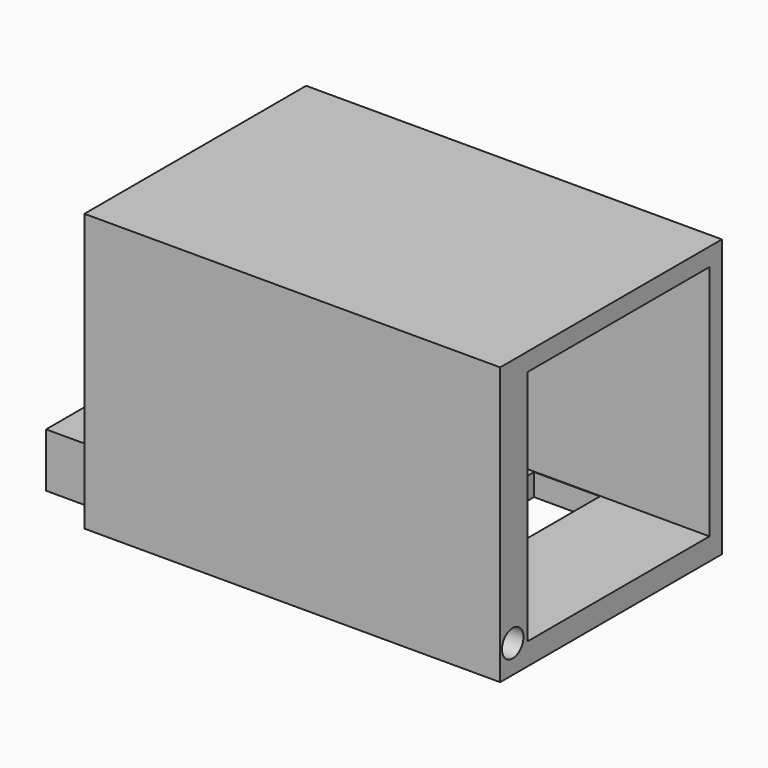
from build123d import *

# Parameters (mm, degrees)
F0_W         = 17.1955762447
F0_H         = 101.6
F0_W_2       = 121.0433589118
F0_W_3       = 14.1610648435
F1_DEPTH     = 101.6
F2_R         = 4.9213514136
F3_DEPTH     = 164.846
F4_W         = 24.1568293422
F4_H         = 84.1714516282
F5_DEPTH     = 19.812
F6_TEXT_SIZE = 13.509515499
F7_DEPTH     = 2.032
F8_DEPTH     = 111.506
F9_W         = 83.3843462169
F9_H         = 86.921655573
F10_DEPTH    = 139.954


# Not quite as in the source:
# - Text() gives the source's letters only with a copy of the font that has no kerning and outlines rounded to 1/6400 em; it was checked with that copy


with BuildPart() as f1:
    # F0 (on Top) → F1 (new body)
    with BuildSketch(Plane.XY):
        with Locations((73.6461340337, 72.8689902046)):
            Rectangle(F0_W, F0_H)
        with Locations((-9.634398388, 72.8689902046)):
            Rectangle(F0_W_2, F0_H)
        with Locations((57.9678134896, 72.8689902046)):
            Rectangle(F0_W_3, F0_H)
    extrude(amount=F1_DEPTH)

    # F2 (on face) → F3 (cut)
    with BuildSketch(Plane(origin=(-70.1560778439, 0, 0), x_dir=(0, -1, 0), z_dir=(-1, 0, 0))):
        with Locations((-27.8169699013, 10.2606434375)):
            Circle(F2_R)
    extrude(amount=-F3_DEPTH, mode=Mode.SUBTRACT)

    # F4 (on face) → F5 (cut)
    with BuildSketch(Plane(origin=(0, 0, 0), x_dir=(1, 0, 0), z_dir=(0, 0, -1))):
        with Locations((30.1983924583, -75.633931905)):
            Rectangle(F4_W, F4_H)
    extrude(amount=-F5_DEPTH, mode=Mode.SUBTRACT)

    # F6 (on face) → F7 (join)
    with BuildSketch(Plane(origin=(0, 0, 0), x_dir=(1, 0, 0), z_dir=(0, 0, -1))):
        with Locations((-66.122502749, -117.7196577191)):
            Text('NIGHTCORE', F6_TEXT_SIZE, font='Open Sans', text_align=(TextAlign.LEFT, TextAlign.BOTTOM))
    extrude(amount=F7_DEPTH)

    # F8 (add): a face of the model
    f8_faces = [f1.faces().sort_by_distance(p)[0] for p in [
        (18.1199777871, 75.633931905, 9.906),
    ]]
    extrude(f8_faces, amount=-F8_DEPTH)

    # F9 (on face) → F10 (cut)
    with BuildSketch(Plane.YZ.offset(82.2439221561)):
        with Locations((76.2837324291, 51.5461224131)):
            Rectangle(F9_W, F9_H)
    extrude(amount=-F10_DEPTH, mode=Mode.SUBTRACT)


solid = f1.part
